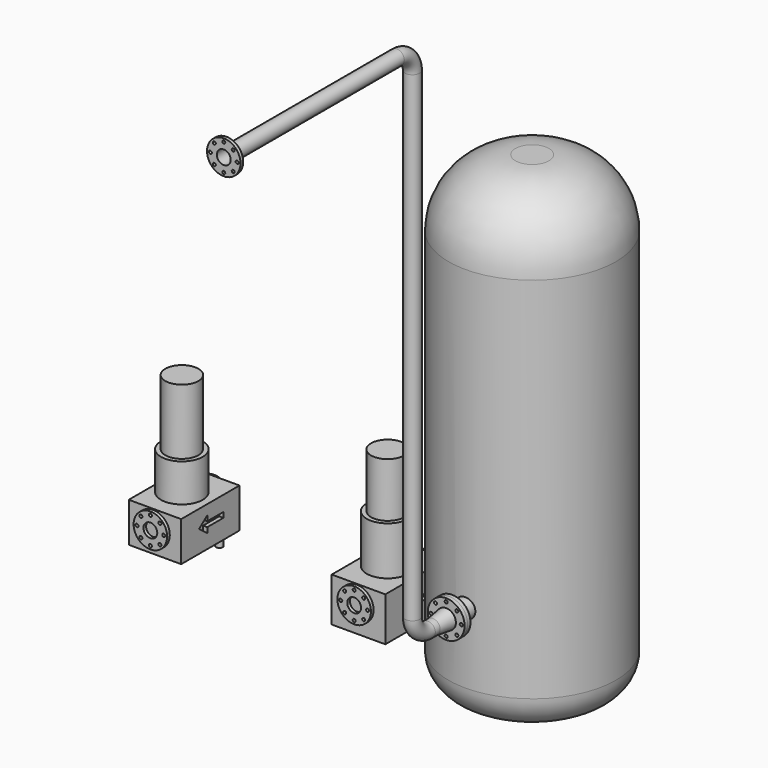
from build123d import *

# Parameters (mm, degrees)
F0_W           = 313
F0_H           = 475
F1_DEPTH       = 853
F5_W           = 313
F5_H           = 236.8338406086
F5_R           = 100
F5_R_2         = 9
F5_R_3         = 41.25
F6_DEPTH       = 20
F7_W           = 313
F7_H           = 236.8338406086
F7_R           = 100
F7_R_2         = 9
F7_R_3         = 41.25
F8_DEPTH       = 20
F10_DEPTH      = 25
F0_W_2         = 320
F0_H_2         = 500
F11_DEPTH      = 876
F15_W          = 320
F15_H          = 262.7112567425
F15_R          = 100
F15_R_2        = 9
F15_R_3        = 41.25
F16_DEPTH      = 20
F17_W          = 320
F17_H          = 262.7112567425
F17_R          = 100
F17_R_2        = 9
F17_R_3        = 41.25
F18_DEPTH      = 20
F20_DEPTH      = 25
F21_R          = 20.2139532789
F22_DEPTH      = 60
F23_R          = 20.2139532789
F24_DEPTH      = 60
F25_R          = 500
F26_DEPTH      = 2800
F27_R          = 400
F28_R          = 200
F30_R          = 58
F30_R_2        = 54.8
F31_DEPTH      = 98
F31_DEPTH_BACK = 20
F32_R          = 110
F32_R_2        = 9
F32_R_3        = 58
F32_R_4        = 57.15
F32_R_5        = 54.8
F33_DEPTH      = 22
F34_DEPTH      = 22
F42_FACE_R     = 44.45
F42_FACE_R_2   = 41.2207572157
F44_R          = 100
F44_R_2        = 9
F44_R_3        = 45.25
F44_R_4        = 44.45
F44_R_5        = 41.2207572157
F45_DEPTH      = 20


with BuildPart() as f1:
    # F0 (on Top) → F1 (new body)
    with BuildSketch(Plane.XY):
        with Locations((-679.8052274053, -123.588575668)):
            Rectangle(F0_W, F0_H)
    extrude(amount=F1_DEPTH)

    # F3 (on offset) → F4 (revolve, cut)
    with BuildSketch(Plane.YZ.offset(-691.3052274053)):
        Polygon((558.0337643623, 853), (-27.088575668, 853), (-27.088575668, 463), (-1.088575668, 463), (-1.088575668, 236.8338406086), (113.911424332, 236.8338406086), (558.0337643623, 236.8338406086), align=None)
    revolve(axis=Axis((-691.3052274053, -126.088575668, 417.7174642682), (0, 0, -1)), mode=Mode.SUBTRACT)

    # F5 (on face) → F6 (cut)
    with BuildSketch(Plane.XZ.offset(361.088575668)):
        with Locations((-679.8052274053, 118.4169203043)):
            Rectangle(F5_W, F5_H)
        with Locations((-691.3052274053, 131)):
            Circle(F5_R, mode=Mode.SUBTRACT)
        with Locations((-747.8737699002, 187.5685424949)):
            Circle(F5_R_2)
        with Locations((-691.3052274053, 211)):
            Circle(F5_R_2)
        with Locations((-634.7366849104, 187.5685424949)):
            Circle(F5_R_2)
        with Locations((-611.3052274053, 131)):
            Circle(F5_R_2)
        with Locations((-634.7366849104, 74.4314575051)):
            Circle(F5_R_2)
        with Locations((-691.3052274053, 51)):
            Circle(F5_R_2)
        with Locations((-747.8737699002, 74.4314575051)):
            Circle(F5_R_2)
        with Locations((-771.3052274053, 131)):
            Circle(F5_R_2)
        with Locations((-691.3052274053, 131)):
            Circle(F5_R_3)
    extrude(amount=-F6_DEPTH, mode=Mode.SUBTRACT)

    # F7 (on face) → F8 (cut)
    with BuildSketch(Plane(origin=(0, 113.911424332, 0), x_dir=(-1, 0, 0), z_dir=(0, 1, 0))):
        with Locations((679.8052274053, 118.4169203043)):
            Rectangle(F7_W, F7_H)
        with Locations((691.3052274053, 131)):
            Circle(F7_R, mode=Mode.SUBTRACT)
        with Locations((691.3052274053, 211)):
            Circle(F7_R_2)
        with Locations((747.8737699002, 187.5685424949)):
            Circle(F7_R_2)
        with Locations((634.7366849104, 187.5685424949)):
            Circle(F7_R_2)
        with Locations((611.3052274053, 131)):
            Circle(F7_R_2)
        with Locations((634.7366849104, 74.4314575051)):
            Circle(F7_R_2)
        with Locations((691.3052274053, 51)):
            Circle(F7_R_2)
        with Locations((747.8737699002, 74.4314575051)):
            Circle(F7_R_2)
        with Locations((771.3052274053, 131)):
            Circle(F7_R_2)
        with Locations((691.3052274053, 131)):
            Circle(F7_R_3)
    extrude(amount=-F8_DEPTH, mode=Mode.SUBTRACT)

    # F9 (on face) → F10 (cut)
    with BuildSketch(Plane.YZ.offset(-523.3052274053)):
        Polygon((-207.5311243534, 131), (-26.3047590852, 131), (-26.3047590852, 146.565469861), (-146.3811099529, 146.565469861), (-146.3811099529, 177.6963797808), align=None)
        Polygon((-26.3047590852, 115.434530139), (-26.3047590852, 131), (-207.5311243534, 131), (-146.3811099529, 84.3036202192), (-146.3811099529, 115.434530139), align=None)
    extrude(amount=-F10_DEPTH, mode=Mode.SUBTRACT)

    # F23 (on face) → F24 (join)
    with BuildSketch(Plane(origin=(0, 0, 0), x_dir=(1, 0, 0), z_dir=(0, 0, -1))):
        with BuildLine():
            ThreePointArc((-691.3052274053, 231.3025289469), (-711.5191806842, 211.088575668), (-691.3052274053, 190.8746223891))
            Line((-691.3052274053, 190.8746223891), (-691.3052274053, 231.3025289469))
        make_face()
        with BuildLine():
            Line((-691.3052274053, 231.3025289469), (-691.3052274053, 190.8746223891))
            ThreePointArc((-691.3052274053, 190.8746223891), (-677.0118039672, 196.7951522299), (-671.0912741264, 211.088575668))
            ThreePointArc((-671.0912741264, 211.088575668), (-677.0118039672, 225.3819991061), (-691.3052274053, 231.3025289469))
        make_face()
        with Locations((-571.3052274053, -3.911424332)):
            Circle(F23_R)
        with Locations((-811.3052274053, -3.911424332)):
            Circle(F23_R)
    extrude(amount=F24_DEPTH)


with BuildPart() as f11:
    # F0 (on Top) → F11 (new body)
    with BuildSketch(Plane.XY):
        with Locations((565.2615959699, -148.3504819324)):
            Rectangle(F0_W_2, F0_H_2)
    extrude(amount=F11_DEPTH)

    # F13 (on offset) → F14 (revolve, cut)
    with BuildSketch(Plane.YZ.offset(555.2615959699)):
        Polygon((461.9782333622, 894.1965103149), (-49.3504819324, 894.1965103149), (-49.3504819324, 551.677107811), (-23.3504819324, 551.677107811), (-23.3504819324, 262.7112567425), (461.9782333622, 262.7112567425), align=None)
    revolve(axis=Axis((555.2615959699, -148.3504819324, 380.9752613306), (0, 0, -1)), mode=Mode.SUBTRACT)

    # F15 (on face) → F16 (cut)
    with BuildSketch(Plane.XZ.offset(398.3504819324)):
        with Locations((565.2615959699, 131.3556283712)):
            Rectangle(F15_W, F15_H)
        with Locations((555.2615959699, 158)):
            Circle(F15_R, mode=Mode.SUBTRACT)
        with Locations((498.693053475, 214.5685424949)):
            Circle(F15_R_2)
        with Locations((555.2615959699, 238)):
            Circle(F15_R_2)
        with Locations((611.8301384649, 214.5685424949)):
            Circle(F15_R_2)
        with Locations((635.2615959699, 158)):
            Circle(F15_R_2)
        with Locations((555.2615959699, 158)):
            Circle(F15_R_3)
        with Locations((611.8301384649, 101.4314575051)):
            Circle(F15_R_2)
        with Locations((555.2615959699, 78)):
            Circle(F15_R_2)
        with Locations((498.693053475, 101.4314575051)):
            Circle(F15_R_2)
        with Locations((475.2615959699, 158)):
            Circle(F15_R_2)
    extrude(amount=-F16_DEPTH, mode=Mode.SUBTRACT)

    # F17 (on face) → F18 (cut)
    with BuildSketch(Plane(origin=(0, 101.6495180676, 0), x_dir=(-1, 0, 0), z_dir=(0, 1, 0))):
        with Locations((-565.2615959699, 131.3556283712)):
            Rectangle(F17_W, F17_H)
        with Locations((-555.2615959699, 158)):
            Circle(F17_R, mode=Mode.SUBTRACT)
        with Locations((-555.2615959699, 238)):
            Circle(F17_R_2)
        with Locations((-498.693053475, 214.5685424949)):
            Circle(F17_R_2)
        with Locations((-498.693053475, 101.4314575051)):
            Circle(F17_R_2)
        with Locations((-555.2615959699, 158)):
            Circle(F17_R_3)
        with Locations((-611.8301384649, 214.5685424949)):
            Circle(F17_R_2)
        with Locations((-635.2615959699, 158)):
            Circle(F17_R_2)
        with Locations((-611.8301384649, 101.4314575051)):
            Circle(F17_R_2)
        with Locations((-555.2615959699, 78)):
            Circle(F17_R_2)
        with Locations((-475.2615959699, 158)):
            Circle(F17_R_2)
    extrude(amount=-F18_DEPTH, mode=Mode.SUBTRACT)

    # F19 (on face) → F20 (cut)
    with BuildSketch(Plane.YZ.offset(725.2615959699)):
        Polygon((-244.788691976, 131.3556283712), (-63.5623267078, 131.3556283712), (-63.5623267078, 146.9210982323), (-183.6386775756, 146.9210982323), (-183.6386775756, 178.052008152), align=None)
        Polygon((-63.5623267078, 115.7901585102), (-63.5623267078, 131.3556283712), (-244.788691976, 131.3556283712), (-183.6386775756, 84.6592485905), (-183.6386775756, 115.7901585102), align=None)
    extrude(amount=-F20_DEPTH, mode=Mode.SUBTRACT)

    # F21 (on face) → F22 (join)
    with BuildSketch(Plane.XY):
        with BuildLine():
            ThreePointArc((555.2615959699, -213.1365286535), (535.047642691, -233.3504819324), (555.2615959699, -253.5644352113))
            Line((555.2615959699, -253.5644352113), (555.2615959699, -213.1365286535))
        make_face()
        with BuildLine():
            Line((555.2615959699, -213.1365286535), (555.2615959699, -253.5644352113))
            ThreePointArc((555.2615959699, -253.5644352113), (569.555019408, -247.6439053705), (575.4755492488, -233.3504819324))
            ThreePointArc((575.4755492488, -233.3504819324), (569.555019408, -219.0570584943), (555.2615959699, -213.1365286535))
        make_face()
        with Locations((680.2615959699, -18.3504819324)):
            Circle(F21_R)
        with Locations((430.2615959699, -18.3504819324)):
            Circle(F21_R)
    extrude(amount=-F22_DEPTH)


with BuildPart() as f26:
    # F25 (on Top) → F26 (new body)
    with BuildSketch(Plane.XY):
        with Locations((1531.4964056015, -290.0888025761)):
            Circle(F25_R)
    extrude(amount=F26_DEPTH)

    # F27
    f27_edges = [f26.edges().sort_by_distance(p)[0] for p in [
        (1031.496406, -290.088803, 2800),
    ]]
    fillet(f27_edges, radius=F27_R)

    # F28
    f28_edges = [f26.edges().sort_by_distance(p)[0] for p in [
        (1031.496406, -290.088803, 0),
    ]]
    fillet(f28_edges, radius=F28_R)

    # F30 (on line) → F31 (join, two sides)
    with BuildSketch(Plane.XZ.offset(790.0888025761)) as f31_sk:
        with Locations((1531.4964056015, 620)):
            Circle(F30_R)
        with Locations((1531.4964056015, 620)):
            Circle(F30_R_2, mode=Mode.SUBTRACT)
    extrude(amount=F31_DEPTH)
    extrude(f31_sk.sketch, amount=-F31_DEPTH_BACK)

    # F32 (on face) → F33 (join)
    with BuildSketch(Plane.XZ.offset(888.0888025761)):
        with Locations((1531.4964056015, 620)):
            Circle(F32_R)
        with Locations((1467.8567952947, 556.3603896932)):
            Circle(F32_R_2, mode=Mode.SUBTRACT)
        with Locations((1531.4964056015, 530)):
            Circle(F32_R_2, mode=Mode.SUBTRACT)
        with Locations((1595.1360159083, 556.3603896932)):
            Circle(F32_R_2, mode=Mode.SUBTRACT)
        with Locations((1441.4964056015, 620)):
            Circle(F32_R_2, mode=Mode.SUBTRACT)
        with Locations((1467.8567952947, 683.6396103068)):
            Circle(F32_R_2, mode=Mode.SUBTRACT)
        with Locations((1531.4964056015, 620)):
            Circle(F32_R_3, mode=Mode.SUBTRACT)
        with Locations((1621.4964056015, 620)):
            Circle(F32_R_2, mode=Mode.SUBTRACT)
        with Locations((1531.4964056015, 710)):
            Circle(F32_R_2, mode=Mode.SUBTRACT)
        with Locations((1595.1360159083, 683.6396103068)):
            Circle(F32_R_2, mode=Mode.SUBTRACT)
        with Locations((1531.4964056015, 620)):
            Circle(F32_R_3)
        with Locations((1531.4964056015, 620)):
            Circle(F32_R_4, mode=Mode.SUBTRACT)
        with Locations((1531.4964056015, 620)):
            Circle(F32_R_4)
        with Locations((1531.4964056015, 620)):
            Circle(F32_R_5, mode=Mode.SUBTRACT)
    extrude(amount=F33_DEPTH)


with BuildPart() as f34:
    # F34 (new): a face of the model
    f34_faces = [f26.part.faces().sort_by_distance(p)[0] for p in [
        (1424.6076754387, -910.0888025761, 620),
    ]]
    extrude(f34_faces, amount=F34_DEPTH)

    # F41 (on plane+point) → F42 (revolve)
    with BuildSketch(Plane.YZ.offset(1531.4964056015)):
        Polygon((-1032.0888025761, 661.2207572157), (-932.0888025761, 674.7707572157), (-932.0888025761, 674.8), (-932.0888025761, 678), (-1032.0888025761, 664.45), align=None)
    revolve(axis=Axis((1531.4964056015, -1000.1295310259, 620), (0, -1, 0)))

    # F43: sweep along a path in F43_path
    with BuildLine(Plane(origin=(1531.4964056015, -1032.0888025761, 620), x_dir=(0, 1, 0), z_dir=(-1, 0, 0))) as f43_path:
        Line((0, 0), (-36.0814568996, 0))
        ThreePointArc((-36.0814568996, 0), (-118.1058435173, -33.9756133824), (-152.0814568996, -116))
        Line((-152.0814568996, -116), (-152.0814568996, -2986))
        ThreePointArc((-152.0814568996, -2986), (-186.057070282, -3068.0243866176), (-268.0814568996, -3102))
        Line((-268.0814568996, -3102), (-283.3219306469, -3102))
        Line((-283.3219306469, -3102), (-1559.7192018032, -3102))
    # F42_face (on face) → F43 (sweep)
    with BuildSketch(Plane(origin=(1531.4964056015, -1032.0888025761, 620), x_dir=(1, 0, 0), z_dir=(0, -1, 0))):
        Circle(F42_FACE_R)
        Circle(F42_FACE_R_2, mode=Mode.SUBTRACT)
    sweep(path=f43_path.line)

    # F44 (on face) → F45 (join)
    with BuildSketch(Plane.XZ.offset(2591.8080043793)):
        with Locations((1531.4964056015, 3722)):
            Circle(F44_R)
        with Locations((1474.9278631066, 3665.4314575051)):
            Circle(F44_R_2, mode=Mode.SUBTRACT)
        with Locations((1531.4964056015, 3642)):
            Circle(F44_R_2, mode=Mode.SUBTRACT)
        with Locations((1588.0649480964, 3665.4314575051)):
            Circle(F44_R_2, mode=Mode.SUBTRACT)
        with Locations((1451.4964056015, 3722)):
            Circle(F44_R_2, mode=Mode.SUBTRACT)
        with Locations((1474.9278631066, 3778.5685424949)):
            Circle(F44_R_2, mode=Mode.SUBTRACT)
        with Locations((1531.4964056015, 3802)):
            Circle(F44_R_2, mode=Mode.SUBTRACT)
        with Locations((1531.4964056015, 3722)):
            Circle(F44_R_3, mode=Mode.SUBTRACT)
        with Locations((1611.4964056015, 3722)):
            Circle(F44_R_2, mode=Mode.SUBTRACT)
        with Locations((1588.0649480964, 3778.5685424949)):
            Circle(F44_R_2, mode=Mode.SUBTRACT)
        with Locations((1531.4964056015, 3722)):
            Circle(F44_R_3)
        with Locations((1531.4964056015, 3722)):
            Circle(F44_R_4, mode=Mode.SUBTRACT)
        with Locations((1531.4964056015, 3722)):
            Circle(F44_R_4)
        with Locations((1531.4964056015, 3722)):
            Circle(F44_R_5, mode=Mode.SUBTRACT)
    extrude(amount=-F45_DEPTH)


solid = Compound([f1.part, f11.part, f26.part, f34.part])
